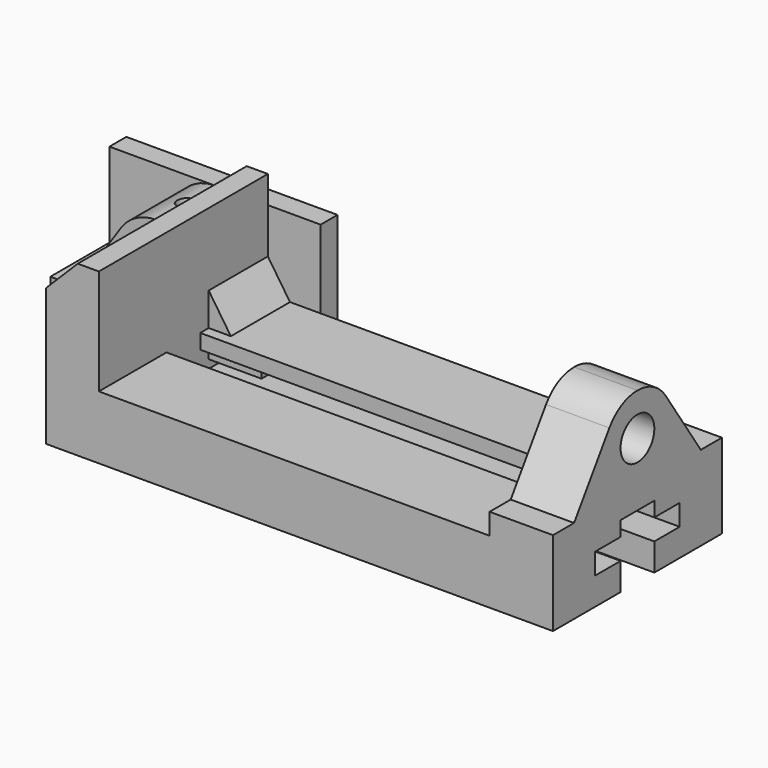
from build123d import *

# Parameters (mm, degrees)
F1_DEPTH  = 127
F2_SIZE2  = 19.05
F2_SIZE   = 19.05
F4_DEPTH  = 50.8
F5_R      = 12.7
F6_DEPTH  = 50.8
F8_DEPTH  = 273.05
F10_DEPTH = 44.45
F11_R     = 12.7
F12_DEPTH = 44.45
F13_W     = 127
F13_H     = 85.09
F14_DEPTH = 12.7
F16_DEPTH = 12.7
F18_R     = 5.08
F19_DEPTH = 25.4


with BuildPart() as f1:
    # F0 (on Front) → F1 (new body)
    with BuildSketch(Plane.XZ):
        Polygon((0, 101.6), (0, 0), (304.8, 0), (304.8, 101.6), (266.7, 101.6), (266.7, 38.1), (31.75, 38.1), (31.75, 101.6), align=None)
    extrude(amount=F1_DEPTH)

    # F2
    f2_edges = [f1.edges().sort_by_distance(p)[0] for p in [
        (0, -63.5, 101.6),
    ]]
    chamfer(f2_edges, length=F2_SIZE, length2=F2_SIZE2)

    # F3 (on face) → F4 (cut)
    with BuildSketch(Plane.YZ.offset(304.8)):
        with BuildLine():
            Line((-127, 101.6), (-127, 50.8))
            Line((-127, 50.8), (-111.125, 50.8))
            Line((-111.125, 50.8), (-84.5934256055, 90.3501730104))
            ThreePointArc((-84.5934256055, 90.3501730104), (-75.4529411765, 98.6117647059), (-63.5, 101.6))
            Line((-63.5, 101.6), (-127, 101.6))
        make_face()
        with BuildLine():
            Line((0, 101.6), (-63.5, 101.6))
            ThreePointArc((-63.5, 101.6), (-51.5470588235, 98.6117647059), (-42.4065743945, 90.3501730104))
            Line((-42.4065743945, 90.3501730104), (-15.875, 50.8))
            Line((-15.875, 50.8), (0, 50.8))
            Line((0, 50.8), (0, 101.6))
        make_face()
    extrude(amount=-F4_DEPTH, mode=Mode.SUBTRACT)

    # F5 (on face) → F6 (cut)
    with BuildSketch(Plane.YZ.offset(304.8)):
        with Locations((-63.5, 76.2)):
            Circle(F5_R)
    extrude(amount=-F6_DEPTH, mode=Mode.SUBTRACT)

    # F7 (on face) → F8 (cut, through all)
    with BuildSketch(Plane.YZ.offset(304.8)):
        Polygon((-76.2, 16.51), (-76.2, 0), (-50.8, 0), (-50.8, 16.51), (-31.75, 16.51), (-31.75, 29.21), (-50.8, 29.21), (-50.8, 38.1), (-76.2, 38.1), (-76.2, 29.21), (-95.25, 29.21), (-95.25, 16.51), align=None)
    extrude(amount=-F8_DEPTH, mode=Mode.SUBTRACT)


with BuildPart() as f10:
    # F9 (on Front) → F10 (new body)
    with BuildSketch(Plane.XZ):
        with BuildLine():
            Line((-31.75, 12.7), (-31.75, 0))
            Line((-31.75, 0), (31.75, 0))
            Line((31.75, 0), (31.75, 12.7))
            Line((31.75, 12.7), (12.7, 12.7))
            Line((12.7, 12.7), (12.7, 21.59))
            Line((12.7, 21.59), (63.5, 21.59))
            Line((63.5, 21.59), (63.5, 34.29))
            Line((63.5, 34.29), (47.625, 34.29))
            Line((47.625, 34.29), (21.0934256055, 73.8401730104))
            ThreePointArc((21.0934256055, 73.8401730104), (0, 85.09), (-21.0934256055, 73.8401730104))
            Line((-21.0934256055, 73.8401730104), (-47.625, 34.29))
            Line((-47.625, 34.29), (-63.5, 34.29))
            Line((-63.5, 34.29), (-63.5, 21.59))
            Line((-63.5, 21.59), (-12.7, 21.59))
            Line((-12.7, 21.59), (-12.7, 12.7))
            Line((-12.7, 12.7), (-31.75, 12.7))
        make_face()
    extrude(amount=F10_DEPTH)

    # F11 (on face) → F12 (cut)
    with BuildSketch(Plane.XZ.offset(44.45)):
        with Locations((0, 59.69)):
            Circle(F11_R)
    extrude(amount=-F12_DEPTH, mode=Mode.SUBTRACT)

    # F13 (on face) → F14 (join)
    with BuildSketch(Plane(origin=(0, 0, 0), x_dir=(-1, 0, 0), z_dir=(0, 1, 0))):
        with Locations((0, 42.545)):
            Rectangle(F13_W, F13_H)
    extrude(amount=F14_DEPTH)

    # F15 (on face) → F16 (cut)
    with BuildSketch(Plane(origin=(0, 12.7, 0), x_dir=(-1, 0, 0), z_dir=(0, 1, 0))):
        Polygon((-63.5, 21.59), (-63.5, 0), (-31.75, 0), (-31.75, 12.7), (-12.7, 12.7), (-12.7, 21.59), align=None)
        Polygon((63.5, 21.59), (12.7, 21.59), (12.7, 12.7), (31.75, 12.7), (31.75, 0), (63.5, 0), align=None)
    extrude(amount=-F16_DEPTH, mode=Mode.SUBTRACT)

    # F18 (on offset) → F19 (cut)
    with BuildSketch(Plane.XY.offset(85.09)):
        with Locations((0, -22.225)):
            Circle(F18_R)
    extrude(amount=-F19_DEPTH, mode=Mode.SUBTRACT)


solid = Compound([f1.part, f10.part])
